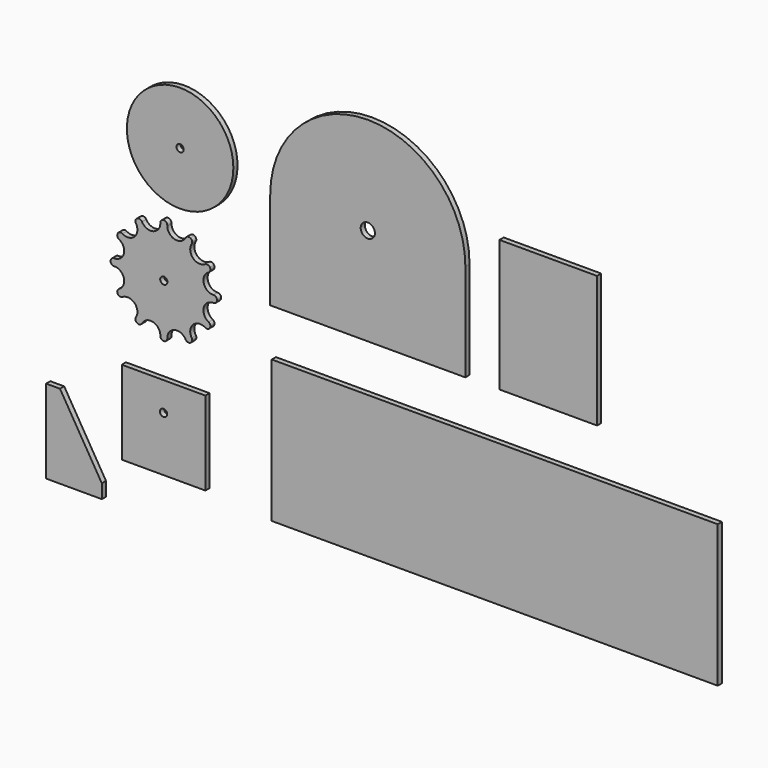
from build123d import *

# Parameters (mm, degrees)
F0_R      = 48.51019
F0_R_2    = 3.302
F1_DEPTH  = 4.7625
F3_DEPTH  = 4.7635
F5_DEPTH  = 4.7625
F6_W      = 406.4
F6_H      = 129.54
F7_DEPTH  = 4.7625
F8_W      = 88.9
F8_H      = 120.015
F9_DEPTH  = 4.7625
F10_W     = 76.2
F10_H     = 38.1
F10_R     = 3.302
F11_DEPTH = 4.7625
F13_DEPTH = 4.7625


with BuildPart() as f1:
    # F0 (on Front) → F1 (new body)
    with BuildSketch(Plane.XZ):
        with Locations((-95.1490104198, 44.2803166807)):
            Circle(F0_R)
        with Locations((-95.1490104198, 44.2803166807)):
            Circle(F0_R_2, mode=Mode.SUBTRACT)
    extrude(amount=F1_DEPTH)


with BuildPart() as f1b:
    # F0 (on Front) → F1, piece 2 (new body)
    with BuildSketch(Plane.XZ):
        with Locations((-110.009752214, -66.7496547103)):
            Circle(F0_R)
        with Locations((-110.009752214, -66.7496547103)):
            Circle(F0_R_2, mode=Mode.SUBTRACT)
    extrude(amount=F1_DEPTH)

    # F2 (on face) → F3 (cut, through all)
    with BuildSketch(Plane.XZ.offset(4.7625)):
        with BuildLine():
            ThreePointArc((-113.184752214, -21.4144647103), (-112.2548162442, -19.16940068), (-110.009752214, -18.2394647103))
            ThreePointArc((-110.009752214, -18.2394647103), (-122.5651132675, -19.8924093511), (-134.264847214, -24.7385978279))
            ThreePointArc((-134.264847214, -24.7385978279), (-131.8555967458, -24.4214139864), (-129.9277165569, -25.9007284849))
            ThreePointArc((-129.9277165569, -25.9007284849), (-129.8851930229, -25.9767722422), (-129.8447720346, -26.0539541551))
            ThreePointArc((-129.8447720346, -26.0539541551), (-119.7676866428, -30.332547645), (-113.1799714423, -21.5886342944))
            ThreePointArc((-113.1799714423, -21.5886342944), (-113.183556796, -21.501582303), (-113.184752214, -21.4144647103))
        make_face()
        with BuildLine():
            ThreePointArc((-85.7546573537, -24.7385977472), (-97.4543912383, -19.8924093302), (-110.009752214, -18.2394647103))
            ThreePointArc((-110.009752214, -18.2394647103), (-107.7646881837, -19.16940068), (-106.834752214, -21.4144647103))
            ThreePointArc((-106.834752214, -21.4144647103), (-106.8359476319, -21.501582303), (-106.8395329856, -21.5886342944))
            ThreePointArc((-106.8395329856, -21.5886342944), (-100.2518177851, -30.332547645), (-90.1747323934, -26.0539541551))
            ThreePointArc((-90.1747323934, -26.0539541551), (-90.134311405, -25.9767722422), (-90.091787871, -25.9007284849))
            ThreePointArc((-90.091787871, -25.9007284849), (-88.1639077601, -24.4214140073), (-85.7546573537, -24.7385977472))
        make_face()
        with BuildLine():
            ThreePointArc((-135.426977871, -29.0757284849), (-135.7441617124, -26.6664780167), (-134.264847214, -24.7385978279))
            ThreePointArc((-134.264847214, -24.7385978279), (-144.3116365196, -32.4477704046), (-152.0208090964, -42.4945597103))
            ThreePointArc((-152.0208090964, -42.4945597103), (-150.0929289075, -41.0152452118), (-147.6836784393, -41.3324290533))
            ThreePointArc((-147.6836784393, -41.3324290533), (-147.6088301, -41.3770231119), (-147.5352335407, -41.423654115))
            ThreePointArc((-147.5352335407, -41.423654115), (-136.6689248504, -40.0904820738), (-135.3357528092, -29.2241733835))
            ThreePointArc((-135.3357528092, -29.2241733835), (-135.3823838123, -29.1505768243), (-135.426977871, -29.0757284849))
        make_face()
        with BuildLine():
            ThreePointArc((-67.9986953552, -42.4945596694), (-75.7078679821, -32.4477703309), (-85.7546573537, -24.7385977472))
            ThreePointArc((-85.7546573537, -24.7385977472), (-84.5925265973, -25.900728415), (-84.167157214, -27.4882284849))
            ThreePointArc((-84.167157214, -27.4882284849), (-84.2753427155, -28.3099789531), (-84.5925265569, -29.0757284849))
            ThreePointArc((-84.5925265569, -29.0757284849), (-84.6371206156, -29.1505768243), (-84.6837516187, -29.2241733835))
            ThreePointArc((-84.6837516187, -29.2241733835), (-83.3505795775, -40.0904820738), (-72.4842708872, -41.423654115))
            ThreePointArc((-72.4842708872, -41.423654115), (-72.410674328, -41.3770231119), (-72.3358259886, -41.3324290533))
            ThreePointArc((-72.3358259886, -41.3324290533), (-69.9265755432, -41.0152452057), (-67.9986953552, -42.4945596694))
        make_face()
        with BuildLine():
            ThreePointArc((-150.8586784393, -46.8316903673), (-152.3379929378, -44.9038101785), (-152.0208090964, -42.4945597103))
            ThreePointArc((-152.0208090964, -42.4945597103), (-156.8669975731, -54.1942936568), (-158.519942214, -66.7496547103))
            ThreePointArc((-158.519942214, -66.7496547103), (-157.5900062442, -64.50459068), (-155.344942214, -63.5746547103))
            ThreePointArc((-155.344942214, -63.5746547103), (-155.2578246213, -63.5758501282), (-155.1707726298, -63.5794354819))
            ThreePointArc((-155.1707726298, -63.5794354819), (-146.4268592793, -56.9917202815), (-150.7054527691, -46.9146348897))
            ThreePointArc((-150.7054527691, -46.9146348897), (-150.782634682, -46.8742139013), (-150.8586784393, -46.8316903673))
        make_face()
        with BuildLine():
            ThreePointArc((-61.499562214, -66.7496547103), (-63.1525068609, -54.1942936339), (-67.9986953552, -42.4945596694))
            ThreePointArc((-67.9986953552, -42.4945596694), (-67.6815114962, -43.2603092193), (-67.5733259886, -44.0820597103))
            ThreePointArc((-67.5733259886, -44.0820597103), (-67.9986953315, -45.6695597103), (-69.1608259886, -46.8316903673))
            ThreePointArc((-69.1608259886, -46.8316903673), (-69.2368697459, -46.8742139013), (-69.3140516588, -46.9146348897))
            ThreePointArc((-69.3140516588, -46.9146348897), (-73.5926451486, -56.9917202815), (-64.8487317981, -63.5794354819))
            ThreePointArc((-64.8487317981, -63.5794354819), (-64.7616798066, -63.5758501282), (-64.674562214, -63.5746547103))
            ThreePointArc((-64.674562214, -63.5746547103), (-62.4294981837, -64.50459068), (-61.499562214, -66.7496547103))
        make_face()
        with BuildLine():
            ThreePointArc((-155.344942214, -69.9246547103), (-157.5900062442, -68.9947187406), (-158.519942214, -66.7496547103))
            ThreePointArc((-158.519942214, -66.7496547103), (-156.8669975731, -79.3050157638), (-152.0208090964, -91.0047497103))
            ThreePointArc((-152.0208090964, -91.0047497103), (-152.3379929378, -88.5954992421), (-150.8586784393, -86.6676190533))
            ThreePointArc((-150.8586784393, -86.6676190533), (-150.782634682, -86.6250955193), (-150.7054527691, -86.5846745309))
            ThreePointArc((-150.7054527691, -86.5846745309), (-146.4268592793, -76.5075891391), (-155.1707726298, -69.9198739387))
            ThreePointArc((-155.1707726298, -69.9198739387), (-155.2578246213, -69.9234592923), (-155.344942214, -69.9246547103))
        make_face()
        with BuildLine():
            ThreePointArc((-67.9986955276, -91.0047500499), (-63.1525069055, -79.3050159532), (-61.499562214, -66.7496547103))
            ThreePointArc((-61.499562214, -66.7496547103), (-62.4294981837, -68.9947187406), (-64.674562214, -69.9246547103))
            ThreePointArc((-64.674562214, -69.9246547103), (-64.7616798066, -69.9234592923), (-64.8487317981, -69.9198739387))
            ThreePointArc((-64.8487317981, -69.9198739387), (-73.5926451486, -76.5075891391), (-69.3140516588, -86.5846745309))
            ThreePointArc((-69.3140516588, -86.5846745309), (-69.2368697459, -86.6250955193), (-69.1608259886, -86.6676190533))
            ThreePointArc((-69.1608259886, -86.6676190533), (-67.9986953315, -87.8297497103), (-67.5733259886, -89.4172497103))
            ThreePointArc((-67.5733259886, -89.4172497103), (-67.6815115408, -90.2390003679), (-67.9986955276, -91.0047500499))
        make_face()
        with BuildLine():
            ThreePointArc((-147.6836784393, -92.1668803673), (-150.0929289075, -92.4840642088), (-152.0208090964, -91.0047497103))
            ThreePointArc((-152.0208090964, -91.0047497103), (-144.3116365196, -101.0515390159), (-134.264847214, -108.7607115927))
            ThreePointArc((-134.264847214, -108.7607115927), (-135.7441617124, -106.8328314039), (-135.426977871, -104.4235809357))
            ThreePointArc((-135.426977871, -104.4235809357), (-135.3823838123, -104.3487325963), (-135.3357528092, -104.2751360371))
            ThreePointArc((-135.3357528092, -104.2751360371), (-136.6689248504, -93.4088273468), (-147.5352335407, -92.0756553056))
            ThreePointArc((-147.5352335407, -92.0756553056), (-147.6088301, -92.1222863087), (-147.6836784393, -92.1668803673))
        make_face()
        with BuildLine():
            ThreePointArc((-85.7546576608, -108.7607118507), (-75.7078682294, -101.051539337), (-67.9986955276, -91.0047500499))
            ThreePointArc((-67.9986955276, -91.0047500499), (-69.9265757098, -92.4840642595), (-72.3358259886, -92.1668803673))
            ThreePointArc((-72.3358259886, -92.1668803673), (-72.410674328, -92.1222863087), (-72.4842708872, -92.0756553056))
            ThreePointArc((-72.4842708872, -92.0756553056), (-83.3505795775, -93.4088273468), (-84.6837516187, -104.2751360371))
            ThreePointArc((-84.6837516187, -104.2751360371), (-84.6371206156, -104.3487325963), (-84.5925265569, -104.4235809357))
            ThreePointArc((-84.5925265569, -104.4235809357), (-84.2753427155, -105.1893304675), (-84.167157214, -106.0110809357))
            ThreePointArc((-84.167157214, -106.0110809357), (-84.5925266859, -107.5985811591), (-85.7546576608, -108.7607118507))
        make_face()
        with BuildLine():
            ThreePointArc((-129.9277165569, -107.5985809357), (-131.8555967458, -109.0778954342), (-134.264847214, -108.7607115927))
            ThreePointArc((-134.264847214, -108.7607115927), (-122.5651132675, -113.6069000695), (-110.009752214, -115.2598447103))
            ThreePointArc((-110.009752214, -115.2598447103), (-112.2548162442, -114.3299087406), (-113.184752214, -112.0848447103))
            ThreePointArc((-113.184752214, -112.0848447103), (-113.183556796, -111.9977271176), (-113.1799714423, -111.9106751262))
            ThreePointArc((-113.1799714423, -111.9106751262), (-119.7676866428, -103.1667617756), (-129.8447720346, -107.4453552655))
            ThreePointArc((-129.8447720346, -107.4453552655), (-129.8851930229, -107.5225371783), (-129.9277165569, -107.5985809357))
        make_face()
        with BuildLine():
            ThreePointArc((-110.009752214, -115.2598447103), (-97.4543914096, -113.6069001363), (-85.7546576608, -108.7607118507))
            ThreePointArc((-85.7546576608, -108.7607118507), (-88.1639079314, -109.0778953674), (-90.091787871, -107.5985809357))
            ThreePointArc((-90.091787871, -107.5985809357), (-90.134311405, -107.5225371783), (-90.1747323934, -107.4453552655))
            ThreePointArc((-90.1747323934, -107.4453552655), (-100.2518177851, -103.1667617756), (-106.8395329856, -111.9106751262))
            ThreePointArc((-106.8395329856, -111.9106751262), (-106.8359476319, -111.9977271176), (-106.834752214, -112.0848447103))
            ThreePointArc((-106.834752214, -112.0848447103), (-107.7646881837, -114.3299087406), (-110.009752214, -115.2598447103))
        make_face()
    extrude(amount=-F3_DEPTH, mode=Mode.SUBTRACT)


with BuildPart() as f5:
    # F4 (on Front) → F5 (new body)
    with BuildSketch(Plane.XZ):
        with BuildLine():
            ThreePointArc((75.8812278509, -55.033158654), (138.7430206984, -28.9949515015), (164.7812278509, 33.866841346))
            Line((164.7812278509, 33.866841346), (82.3582278509, 33.866841346))
            ThreePointArc((82.3582278509, 33.866841346), (75.8812278509, 27.389841346), (69.4042278509, 33.866841346))
            Line((69.4042278509, 33.866841346), (-13.0187721491, 33.866841346))
            ThreePointArc((-13.0187721491, 33.866841346), (13.0194350034, -28.9949515015), (75.8812278509, -55.033158654))
        make_face()
        with BuildLine():
            Line((82.3582278509, 33.866841346), (164.7812278509, 33.866841346))
            ThreePointArc((164.7812278509, 33.866841346), (75.8812278509, 122.766841346), (-13.0187721491, 33.866841346))
            Line((-13.0187721491, 33.866841346), (69.4042278509, 33.866841346))
            ThreePointArc((69.4042278509, 33.866841346), (75.8812278509, 40.343841346), (82.3582278509, 33.866841346))
        make_face()
        with BuildLine():
            ThreePointArc((75.8812278509, -55.033158654), (13.0194350034, -28.9949515015), (-13.0187721491, 33.866841346))
            Line((-13.0187721491, 33.866841346), (-13.0187721491, -55.033158654))
            Line((-13.0187721491, -55.033158654), (75.8812278509, -55.033158654))
        make_face()
        with BuildLine():
            Line((164.7812278509, -55.033158654), (164.7812278509, 33.866841346))
            ThreePointArc((164.7812278509, 33.866841346), (138.7430206984, -28.9949515015), (75.8812278509, -55.033158654))
            Line((75.8812278509, -55.033158654), (164.7812278509, -55.033158654))
        make_face()
    extrude(amount=F5_DEPTH)


with BuildPart() as f7:
    # F6 (on Front) → F7 (new body)
    with BuildSketch(Plane.XZ):
        with Locations((191.5482940495, -162.8059837413)):
            Rectangle(F6_W, F6_H)
    extrude(amount=F7_DEPTH)


with BuildPart() as f9:
    # F8 (on Front) → F9 (new body)
    with BuildSketch(Plane.XZ):
        with Locations((240.3279543638, 5.3869090009)):
            Rectangle(F8_W, F8_H)
    extrude(amount=F9_DEPTH)


with BuildPart() as f11:
    # F10 (on Front) → F11 (new body)
    with BuildSketch(Plane.XZ):
        with Locations((-110.2248355746, -203.7960269928)):
            Rectangle(F10_W, F10_H)
        with BuildLine():
            Line((-148.3248355746, -146.6460269928), (-148.3248355746, -184.7460269928))
            ThreePointArc((-148.3248355746, -184.7460269928), (-137.1656039378, -157.8052586296), (-110.2248355746, -146.6460269928))
            Line((-110.2248355746, -146.6460269928), (-148.3248355746, -146.6460269928))
        make_face()
        with BuildLine():
            ThreePointArc((-110.2248355746, -146.6460269928), (-137.1656039378, -157.8052586296), (-148.3248355746, -184.7460269928))
            Line((-148.3248355746, -184.7460269928), (-72.1248355746, -184.7460269928))
            ThreePointArc((-72.1248355746, -184.7460269928), (-83.2840672114, -157.8052586296), (-110.2248355746, -146.6460269928))
        make_face()
        with Locations((-110.2248355746, -172.9096269928)):
            Circle(F10_R, mode=Mode.SUBTRACT)
        with BuildLine():
            ThreePointArc((-110.2248355746, -146.6460269928), (-83.2840672114, -157.8052586296), (-72.1248355746, -184.7460269928))
            Line((-72.1248355746, -184.7460269928), (-72.1248355746, -146.6460269928))
            Line((-72.1248355746, -146.6460269928), (-110.2248355746, -146.6460269928))
        make_face()
    extrude(amount=F11_DEPTH)


with BuildPart() as f13:
    # F12 (on Front) → F13 (new body)
    with BuildSketch(Plane.XZ):
        Polygon((-217.2843559265, -184.2374587536), (-217.2843559265, -260.4374587536), (-166.4843559265, -260.4374587536), (-166.4843559265, -247.7374587536), (-204.5843559265, -184.2374587536), align=None)
    extrude(amount=F13_DEPTH)


solid = Compound([f1.part, f1b.part, f5.part, f7.part, f9.part, f11.part, f13.part])
